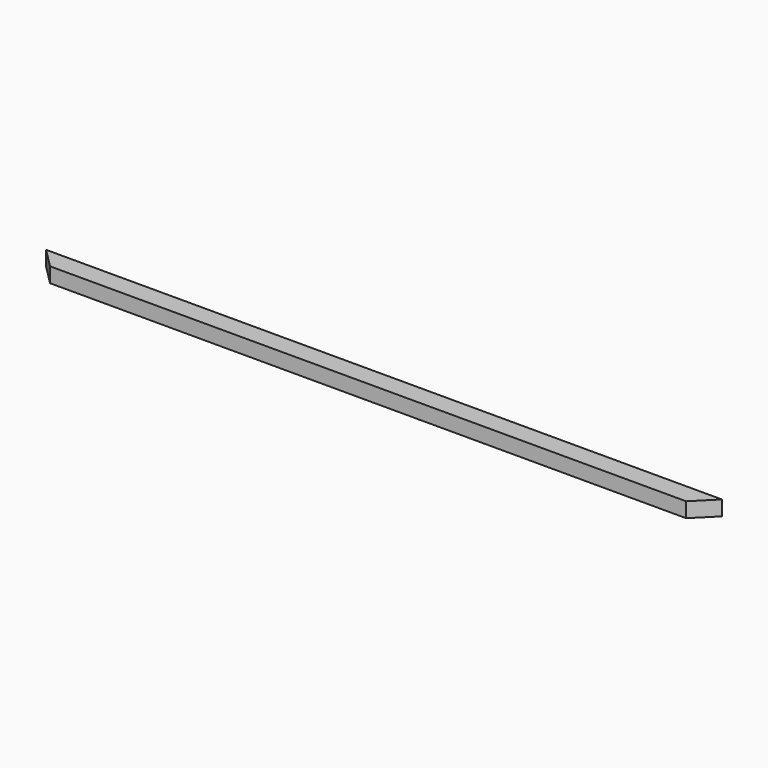
from build123d import *

# Parameters (mm, degrees)
F0_W     = 863.6
F0_H     = 25.4
F1_DEPTH = 19.05
F2_SIZE  = 25.39999


# Not quite as in the source:
# - a fillet or chamfer is up to 0.001 mm smaller than in the source, because OpenCascade refuses the exact size


with BuildPart() as f1:
    # F0 (on Top) → F1 (new body)
    with BuildSketch(Plane.XY):
        with Locations((10.9929144382, -134.3236717459)):
            Rectangle(F0_W, F0_H)
    extrude(amount=F1_DEPTH)

    # F2 (size 25.4 in the source; OpenCascade refuses exactly that, so slightly less here)
    f2_edges = [f1.edges().sort_by_distance(p)[0] for p in [
        (442.792914, -147.023672, 9.525),
        (-420.807086, -147.023672, 9.525),
    ]]
    chamfer(f2_edges, length=F2_SIZE)


solid = f1.part
